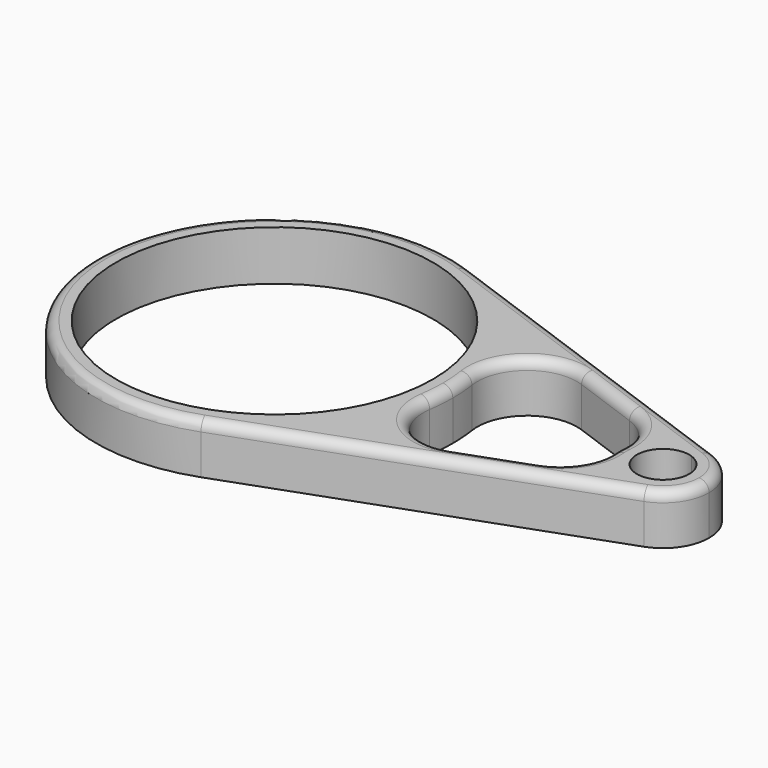
from build123d import *

# Parameters (mm, degrees)
F1_DEPTH = 5
F2_R     = 5
F3_R     = 0.99999


# Not quite as in the source:
# - a fillet or chamfer is up to 0.001 mm smaller than in the source, because OpenCascade refuses the exact size


with BuildPart() as f1:
    # F0 (on Top) → F1 (new body)
    with BuildSketch(Plane.XY):
        with BuildLine():
            ThreePointArc((5.4121153846, -14.9505520655), (-15.9, 0), (5.4121153846, 14.9505520655))
            Line((5.4121153846, 14.9505520655), (13.1430758683, 12.1519363363))
            ThreePointArc((13.1430758683, 12.1519363363), (9.898446583, 14.91411262), (6.0928846154, 16.8311246524))
            ThreePointArc((6.0928846154, 16.8311246524), (-17.9, 0), (6.0928846154, -16.8311246524))
            ThreePointArc((6.0928846154, -16.8311246524), (9.898446583, -14.91411262), (13.1430758683, -12.1519363363))
            Line((13.1430758683, -12.1519363363), (5.4121153846, -14.9505520655))
        make_face()
        with BuildLine():
            ThreePointArc((6.0928846154, 16.8311246524), (9.898446583, 14.91411262), (13.1430758683, 12.1519363363))
            Line((13.1430758683, 12.1519363363), (36.3130060827, 3.76439752))
            ThreePointArc((36.3130060827, 3.76439752), (38.3715715504, 4.5821067953), (40.5742788462, 4.3488241071))
            Line((40.5742788462, 4.3488241071), (6.0928846154, 16.8311246524))
        make_face()
        with BuildLine():
            Line((36.3130060827, -3.76439752), (13.1430758683, -12.1519363363))
            ThreePointArc((13.1430758683, -12.1519363363), (9.898446583, -14.91411262), (6.0928846154, -16.8311246524))
            Line((6.0928846154, -16.8311246524), (40.5742788462, -4.3488241071))
            ThreePointArc((40.5742788462, -4.3488241071), (38.3715715504, -4.5821067953), (36.3130060827, -3.76439752))
        make_face()
        with BuildLine():
            ThreePointArc((40.5742788462, 4.3488241071), (38.3715715504, 4.5821067953), (36.3130060827, 3.76439752))
            Line((36.3130060827, 3.76439752), (39.8935096154, 2.4682515202))
            ThreePointArc((39.8935096154, 2.4682515202), (41.1489634409, 1.507508252), (41.625, 0))
            ThreePointArc((41.625, 0), (41.1489634409, -1.507508252), (39.8935096154, -2.4682515202))
            Line((39.8935096154, -2.4682515202), (36.3130060827, -3.76439752))
            ThreePointArc((36.3130060827, -3.76439752), (38.3715715504, -4.5821067953), (40.5742788462, -4.3488241071))
            ThreePointArc((40.5742788462, -4.3488241071), (42.7862689196, -2.6560859678), (43.625, 0))
            ThreePointArc((43.625, 0), (42.7862689196, 2.6560859678), (40.5742788462, 4.3488241071))
        make_face()
        with BuildLine():
            Line((39.8935096154, 2.4682515202), (36.3130060827, 3.76439752))
            ThreePointArc((36.3130060827, 3.76439752), (34.375, 0), (36.3130060827, -3.76439752))
            Line((36.3130060827, -3.76439752), (39.8935096154, -2.4682515202))
            ThreePointArc((39.8935096154, -2.4682515202), (36.375, 0), (39.8935096154, 2.4682515202))
        make_face()
        with BuildLine():
            ThreePointArc((5.4121153846, 14.9505520655), (13.0165785561, 9.1311928406), (15.9, 0))
            ThreePointArc((15.9, 0), (13.0165785561, -9.1311928406), (5.4121153846, -14.9505520655))
            Line((5.4121153846, -14.9505520655), (13.1430758683, -12.1519363363))
            ThreePointArc((13.1430758683, -12.1519363363), (16.6683991139, -6.5249115687), (17.9, 0))
            ThreePointArc((17.9, 0), (16.6683991139, 6.5249115687), (13.1430758683, 12.1519363363))
            Line((13.1430758683, 12.1519363363), (5.4121153846, 14.9505520655))
        make_face()
    extrude(amount=F1_DEPTH)

    # F2
    f2_edges = [f1.edges().sort_by_distance(p)[0] for p in [
        (36.313006, 3.764398, 2.5),
        (36.313006, -3.764398, 2.5),
        (13.143076, 12.151936, 2.5),
        (13.143076, -12.151936, 2.5),
    ]]
    fillet(f2_edges, radius=F2_R)

    # F3 (radius 1 in the source; OpenCascade refuses exactly that, so slightly less here)
    f3_edges = [f1.edges().sort_by_distance(p)[0] for p in [
        (23.333582, 10.589974, 5),
        (19.479429, 7.262513, 5),
    ]]
    fillet(f3_edges, radius=F3_R)


solid = f1.part
